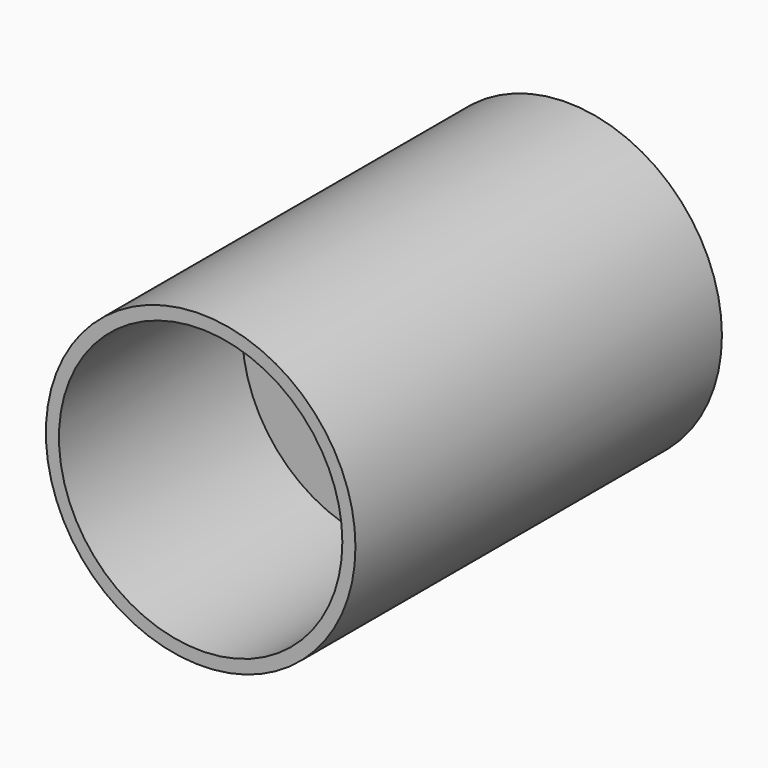
from build123d import *

# Parameters (mm, degrees)
F0_R     = 51.4985
F1_DEPTH = 152.4
F2_R     = 47.1424
F3_DEPTH = 76.2


# Not quite as in the source:
# - a feature names something its author has since deleted; it is built from what else it names


with BuildPart() as f1:
    # F0 (on Front) → F1 (new body)
    with BuildSketch(Plane.XZ):
        Circle(F0_R)
    extrude(amount=F1_DEPTH)

    # F2 (on face) → F3 (cut)
    with BuildSketch(Plane.XZ.offset(152.4)):
        Circle(F2_R)
    extrude(amount=-F3_DEPTH, mode=Mode.SUBTRACT)


solid = f1.part
